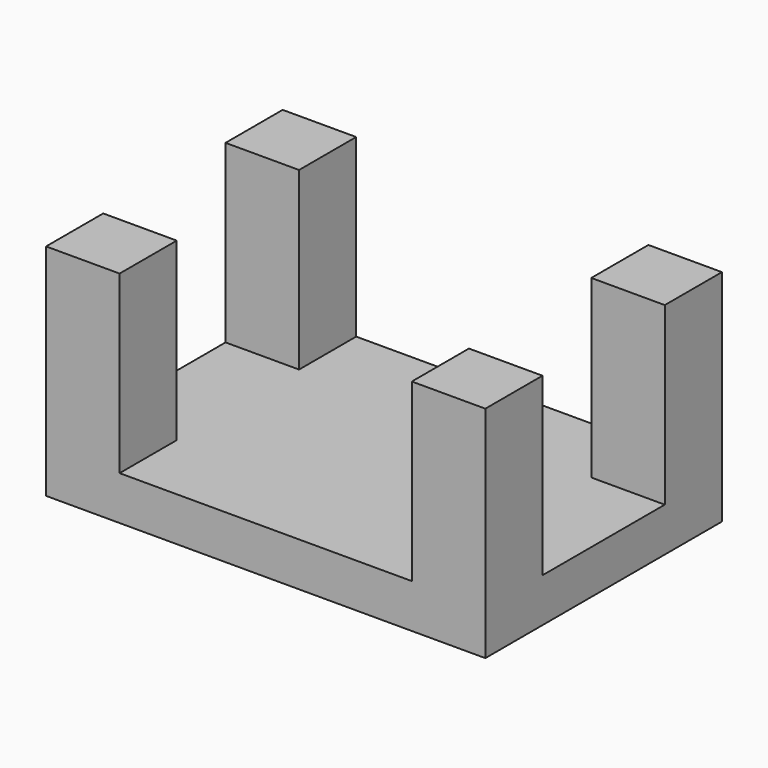
from build123d import *

# Parameters (mm, degrees)
F0_W     = 8.368255198
F0_H     = 8.1290510939
F1_DEPTH = 5
F2_DEPTH = 25


with BuildPart() as f1:
    # F0 (on Top) → F1 (new body)
    with BuildSketch(Plane.XY):
        with Locations((-20.815872401, 12.7671566554)):
            Rectangle(F0_W, F0_H)
        Polygon((16.631744802, 16.8316822024), (-16.631744802, 16.8316822024), (-16.631744802, 8.7026311085), (-25, 8.7026311085), (-25, -8.7026311085), (-16.631744802, -8.7026311085), (-16.631744802, -16.8316822024), (16.631744802, -16.8316822024), (16.631744802, -8.7026311085), (25, -8.7026311085), (25, 8.7026311085), (16.631744802, 8.7026311085), align=None)
        with Locations((20.815872401, 12.7671566554)):
            Rectangle(F0_W, F0_H)
        with Locations((-20.815872401, -12.7671566554)):
            Rectangle(F0_W, F0_H)
        with Locations((20.815872401, -12.7671566554)):
            Rectangle(F0_W, F0_H)
    extrude(amount=F1_DEPTH)

    # F0 (on Top) → F2 (join)
    with BuildSketch(Plane.XY):
        with Locations((20.815872401, 12.7671566554)):
            Rectangle(F0_W, F0_H)
        with Locations((20.815872401, -12.7671566554)):
            Rectangle(F0_W, F0_H)
        with Locations((-20.815872401, -12.7671566554)):
            Rectangle(F0_W, F0_H)
        with Locations((-20.815872401, 12.7671566554)):
            Rectangle(F0_W, F0_H)
    extrude(amount=F2_DEPTH)


solid = f1.part
